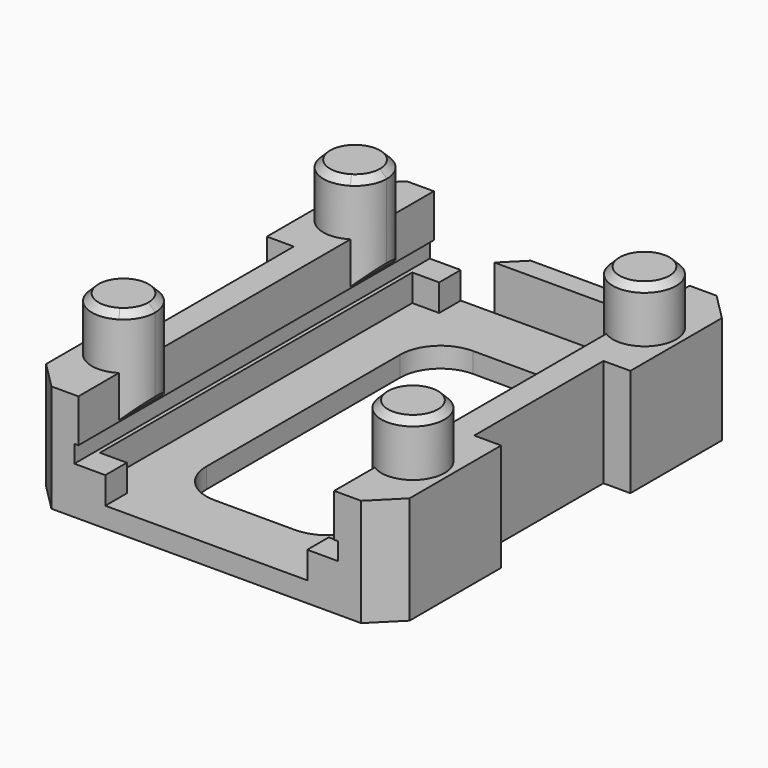
from build123d import *

# Parameters (mm, degrees)
F1_DEPTH       = 1.5
F0_W           = 4
F0_H           = 33
F2_DEPTH       = 8
F3_W           = 33
F3_H           = 1.5
F4_DEPTH       = 0.5
F5_W           = 33
F5_H           = 1.5
F6_DEPTH       = 0.5
F7_W           = 2
F7_H           = 2
F8_DEPTH       = 2
F10_W          = 12
F10_H          = 24
F11_DEPTH      = 1.5
F13_DEPTH      = 25
F14_R          = 3
F9_R           = 2.35
F15_DEPTH      = 4
F16_DEPTH      = 2
F17_DEPTH      = 4
F17_DEPTH_BACK = 2
F18_DEPTH      = 0.2
F19_DEPTH      = 0.2
F20_DEPTH      = 0.2
F21_SIZE       = 0.5
F22_C1_SIZE    = 1.0999
F22_C2_SIZE    = 1.0999
F22_C3_SIZE    = 1.0999
F22_T7_DEPTH   = 9.637652322
F22_S8_R       = 2.35
F22_T9_DEPTH   = 6
F23_DEPTH      = 4.8
F24_SIZE       = 1.49999
F25_SIZE       = 2


# Not quite as in the source:
# - a fillet or chamfer that OpenCascade refuses, or shapes differently, is made with other operations: its cross-section is extruded or revolved along the edge and cut away or added
# - a fillet or chamfer is up to 0.001 mm smaller than in the source, because OpenCascade refuses the exact size


with BuildPart() as f1:
    # F0 (on Top) → F1 (new body)
    with BuildSketch(Plane.XY):
        Polygon((9.5, -16.5), (9.5, 16.5), (5, 16.5), (-5, 16.5), (-9.5, 16.5), (-9.5, -16.5), align=None)
    extrude(amount=F1_DEPTH)

    # F0 (on Top) → F2 (join)
    with BuildSketch(Plane.XY):
        with Locations((-11.5, 0)):
            Rectangle(F0_W, F0_H)
        with Locations((11.5, 0)):
            Rectangle(F0_W, F0_H)
    extrude(amount=F2_DEPTH)

    # F3 (on face) → F4 (cut)
    with BuildSketch(Plane.YZ.offset(-9.5)):
        with Locations((0, 4.25)):
            Rectangle(F3_W, F3_H)
    extrude(amount=-F4_DEPTH, mode=Mode.SUBTRACT)

    # F5 (on face) → F6 (cut)
    with BuildSketch(Plane(origin=(9.5, 0, 0), x_dir=(0, -1, 0), z_dir=(-1, 0, 0))):
        with Locations((0, 4.25)):
            Rectangle(F5_W, F5_H)
    extrude(amount=-F6_DEPTH, mode=Mode.SUBTRACT)

    # F7 (on face) → F8 (join)
    with BuildSketch(Plane.XY.offset(1.5)):
        with Locations((-8.5, 15.5)):
            Rectangle(F7_W, F7_H)
        with Locations((8.5, 15.5)):
            Rectangle(F7_W, F7_H)
        with Locations((8.5, -15.5)):
            Rectangle(F7_W, F7_H)
        with Locations((-8.5, -15.5)):
            Rectangle(F7_W, F7_H)
    extrude(amount=F8_DEPTH)

    # F10 (on face) → F11 (cut)
    with BuildSketch(Plane.XY.offset(1.5)):
        Rectangle(F10_W, F10_H)
    extrude(amount=-F11_DEPTH, mode=Mode.SUBTRACT)

    # F12 (on face) → F13 (cut)
    with BuildSketch(Plane.XY.offset(8)):
        Polygon((13.5, -6), (13.5, 6), (11.5, 6), (11.5, 0), (11.5, -6), align=None)
        Polygon((-11.5, 6), (-13.5, 6), (-13.5, -6), (-11.5, -6), (-11.5, 0), align=None)
    extrude(amount=-F13_DEPTH, mode=Mode.SUBTRACT)

    # F14
    f14_edges = [f1.edges().sort_by_distance(p)[0] for p in [
        (6, 12, 0.75),
        (-6, 12, 0.75),
        (-6, -12, 0.75),
        (6, -12, 0.75),
    ]]
    fillet(f14_edges, radius=F14_R)

    # F9 (on face) → F15 (join)
    with BuildSketch(Plane.XY.offset(8)):
        with BuildLine():
            Line((-9.5, 8.7600251258), (-9.5, 12.7399748742))
            ThreePointArc((-9.5, 12.7399748742), (-13.1, 10.75), (-9.5, 8.7600251258))
        make_face()
        with Locations((10.75, 10.75)):
            Circle(F9_R)
        with BuildLine():
            ThreePointArc((-8.4, -10.75), (-8.6933036199, -9.6131182999), (-9.5, -8.7600251258))
            Line((-9.5, -8.7600251258), (-9.5, -12.7399748742))
            ThreePointArc((-9.5, -12.7399748742), (-8.6933036199, -11.8868817001), (-8.4, -10.75))
        make_face()
        with Locations((10.75, -10.75)):
            Circle(F9_R)
    extrude(amount=F15_DEPTH)

    # F16 (add): faces of the model
    f16_faces = [f1.faces().sort_by_distance(p)[0] for p in [
        (9.0497739869, -10.75, 8),
        (9.0497739869, 10.75, 8),
    ]]
    extrude(f16_faces, amount=F16_DEPTH)

    # F9 (on face) → F17 (join, two sides)
    with BuildSketch(Plane.XY.offset(8)) as f17_sk:
        with BuildLine():
            ThreePointArc((-9.5, 8.7600251258), (-8.6933036199, 9.6131182999), (-8.4, 10.75))
            ThreePointArc((-8.4, 10.75), (-8.6933036199, 11.8868817001), (-9.5, 12.7399748742))
            Line((-9.5, 12.7399748742), (-9.5, 8.7600251258))
        make_face()
        with BuildLine():
            Line((-9.5, -12.7399748742), (-9.5, -8.7600251258))
            ThreePointArc((-9.5, -8.7600251258), (-13.1, -10.75), (-9.5, -12.7399748742))
        make_face()
        with BuildLine():
            ThreePointArc((-8.4, -10.75), (-8.6933036199, -9.6131182999), (-9.5, -8.7600251258))
            Line((-9.5, -8.7600251258), (-9.5, -12.7399748742))
            ThreePointArc((-9.5, -12.7399748742), (-8.6933036199, -11.8868817001), (-8.4, -10.75))
        make_face()
    extrude(amount=F17_DEPTH)
    extrude(f17_sk.sketch, amount=-F17_DEPTH_BACK)

    # F18 (add): faces of the model
    f18_faces = [f1.faces().sort_by_distance(p)[0] for p in [
        (-9.75, 0, 5),
        (9.75, 0, 5),
    ]]
    extrude(f18_faces, amount=F18_DEPTH)

    # F19 (add): a face of the model
    f19_faces = [f1.faces().sort_by_distance(p)[0] for p in [
        (-10, 0, 4.15),
    ]]
    extrude(f19_faces, amount=F19_DEPTH)

    # F20 (add): a face of the model
    f20_faces = [f1.faces().sort_by_distance(p)[0] for p in [
        (10, 0, 4.15),
    ]]
    extrude(f20_faces, amount=F20_DEPTH)

    # F21
    f21_edges = [f1.edges().sort_by_distance(p)[0] for p in [
        (8.4, 10.75, 12),
        (8.4, -10.75, 12),
        (-13.1, -10.75, 12),
        (-13.1, 10.75, 12),
        (-8.4, 10.75, 12),
        (-8.4, -10.75, 12),
    ]]
    chamfer(f21_edges, length=F21_SIZE)

    # F22: chamfer of 1.1 on 4 edges, made by hand

    # F22_c1 (size 1.1 in the source; OpenCascade refuses exactly that, so slightly less here)
    f22_c1_edges = [f1.edges().sort_by_distance(p)[0] for p in [
        (9.5, 10.75, 6),
    ]]
    chamfer(f22_c1_edges, length=F22_C1_SIZE)

    # F22_c2 (size 1.1 in the source; OpenCascade refuses exactly that, so slightly less here)
    f22_c2_edges = [f1.edges().sort_by_distance(p)[0] for p in [
        (9.5, -10.75, 6),
    ]]
    chamfer(f22_c2_edges, length=F22_C2_SIZE)

    # F22_c3 (size 1.1 in the source; OpenCascade refuses exactly that, so slightly less here)
    f22_c3_edges = [f1.edges().sort_by_distance(p)[0] for p in [
        (-9.5, 10.75, 6),
    ]]
    chamfer(f22_c3_edges, length=F22_C3_SIZE)


with BuildPart() as f22_tool5:
    # F22_s6 → F22_t7 (new body)
    with BuildSketch(Plane.XZ.offset(15.568826161)):
        with BuildLine():
            Line((-9.5311126984, 4.8688873016), (-8.3688873016, 6.0311126984))
            Line((-8.3688873016, 6.0311126984), (-8.3688873016, 6.0531126984))
            ThreePointArc((-8.3688873016, 6.0531126984), (-8.9344436508, 6.022), (-9.5, 6.022))
            Line((-9.5, 6.022), (-9.522, 6))
            ThreePointArc((-9.522, 6), (-9.522, 5.4344436508), (-9.5531126984, 4.8688873016))
            Line((-9.5531126984, 4.8688873016), (-9.5311126984, 4.8688873016))
        make_face()
    extrude(amount=-F22_T7_DEPTH)

    # F22_s8 → F22_t9 (intersect, symmetric)
    with BuildSketch(Plane.XY.offset(5.5)):
        with Locations((-10.75, -10.75)):
            Circle(F22_S8_R)
    extrude(amount=F22_T9_DEPTH, both=True, mode=Mode.INTERSECT)


with BuildPart() as f1_1:
    add(f1.part)

    # F22_t4: union F22_tool5
    add(f22_tool5.part)

    # F0 (on Top) → F23 (join, through all)
    with BuildSketch(Plane.XY):
        Polygon((-5, 16.5), (5, 16.5), (5, 18), (0, 18), (-5, 18), align=None)
    extrude(amount=F23_DEPTH)

    # F24 (size 1.5 in the source; OpenCascade refuses exactly that, so slightly less here)
    f24_edges = [f1_1.edges().sort_by_distance(p)[0] for p in [
        (-5, 18, 2.4),
        (5, 18, 2.4),
    ]]
    chamfer(f24_edges, length=F24_SIZE)

    # F25
    f25_edges = [f1_1.edges().sort_by_distance(p)[0] for p in [
        (13.5, -16.5, 4),
        (-13.5, -16.5, 4),
        (13.5, 16.5, 4),
        (-13.5, 16.5, 4),
    ]]
    chamfer(f25_edges, length=F25_SIZE)


solid = f1_1.part
